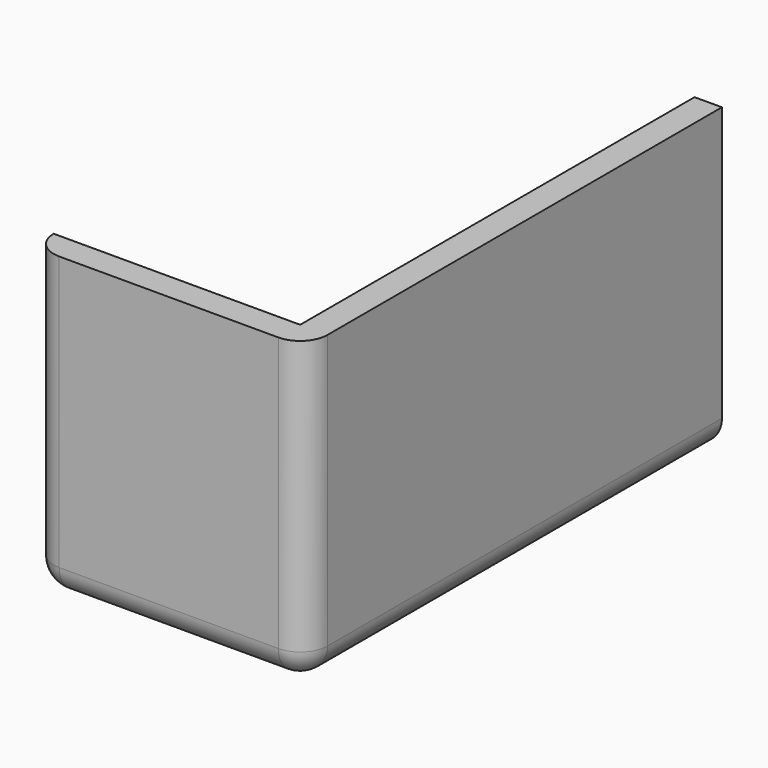
from build123d import *

# Parameters (mm, degrees)
F0_W     = 40
F0_H     = 76
F0_R     = 1.75
F1_DEPTH = 44
F2_W     = 72
F2_H     = 40
F3_DEPTH = 36
F4_R     = 1.5
F5_DEPTH = 4
F6_DEPTH = 4
F7_R     = 3.99999


# Not quite as in the source:
# - a fillet or chamfer is up to 0.001 mm smaller than in the source, because OpenCascade refuses the exact size


with BuildPart() as f1:
    # F0 (on Top) → F1 (new body)
    with BuildSketch(Plane.XY):
        with Locations((20, 38)):
            Rectangle(F0_W, F0_H)
        with Locations((10, 16.5)):
            Circle(F0_R, mode=Mode.SUBTRACT)
        with Locations((10, 63.5)):
            Circle(F0_R, mode=Mode.SUBTRACT)
        with Locations((10, 63.5)):
            Circle(F0_R)
        with Locations((10, 16.5)):
            Circle(F0_R)
    extrude(amount=F1_DEPTH)

    # F2 (on face) → F3 (cut)
    with BuildSketch(Plane(origin=(0, 0, 0), x_dir=(0, -1, 0), z_dir=(-1, 0, 0))):
        with Locations((-40, 24)):
            Rectangle(F2_W, F2_H)
    extrude(amount=-F3_DEPTH, mode=Mode.SUBTRACT)

    # F4 (on face) → F5 (cut)
    with BuildSketch(Plane(origin=(0, 76, 0), x_dir=(-1, 0, 0), z_dir=(0, 1, 0))):
        with BuildLine():
            ThreePointArc((-29.5, 18.5), (-26.6715728753, 19.6715728753), (-25.5, 22.5))
            ThreePointArc((-25.5, 22.5), (-26.6715728753, 25.3284271247), (-29.5, 26.5))
            ThreePointArc((-29.5, 26.5), (-33.5, 22.5), (-29.5, 18.5))
        make_face()
        with Locations((-12, 23.5)):
            Circle(F4_R)
    extrude(amount=-F5_DEPTH, mode=Mode.SUBTRACT)

    # F0 (on Top) → F6 (cut)
    with BuildSketch(Plane.XY):
        with Locations((10, 63.5)):
            Circle(F0_R)
        with Locations((10, 16.5)):
            Circle(F0_R)
    extrude(amount=F6_DEPTH, mode=Mode.SUBTRACT)

    # F7 (radius 4 in the source; OpenCascade refuses exactly that, so slightly less here)
    f7_edges = [f1.edges().sort_by_distance(p)[0] for p in [
        (40, 38, 0),
        (40, 0, 22),
        (0, 0, 22),
        (20, 0, 0),
        (0, 76, 2),
        (0, 38, 0),
    ]]
    fillet(f7_edges, radius=F7_R)


solid = f1.part
